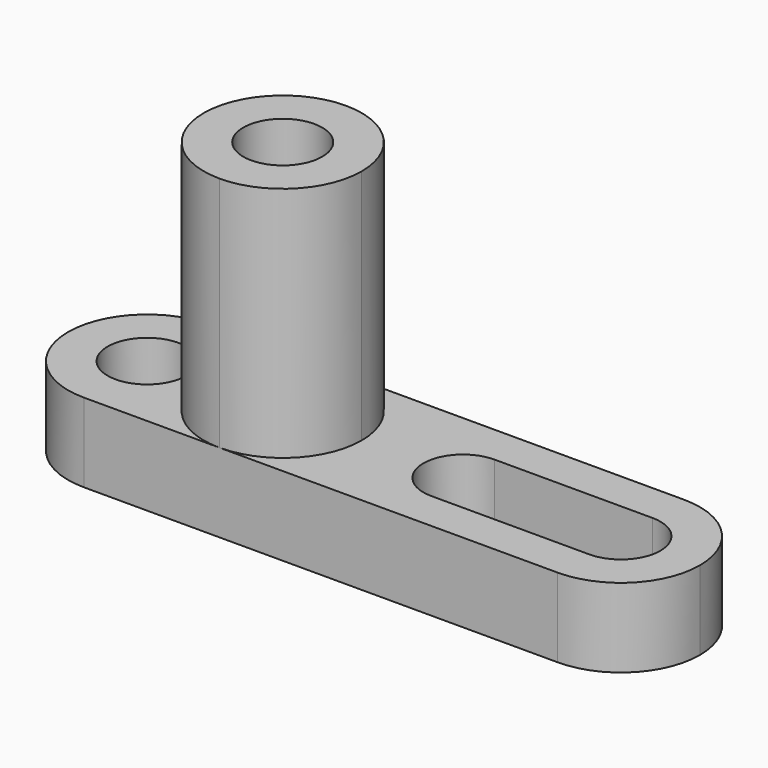
from build123d import *

# Parameters (mm, degrees)
F1_DEPTH = 25.4
F3_DEPTH = 38.1
F4_R     = 6.35
F5_DEPTH = 25.4
F7_DEPTH = 25.4
F8_R     = 6.35
F9_DEPTH = 127


# Not quite as in the source:
# - a feature names something its author has since deleted; it is built from what else it names


with BuildPart() as f1:
    # F0 (on Front) → F1 (new body)
    with BuildSketch(Plane.XZ):
        Polygon((-21.8179498348, 12.7), (-21.8179498348, 0), (79.7820501652, 0), (79.7820501652, 12.7), (25.4, 12.7), (25.4, 50.8), (0, 50.8), (0, 12.7), align=None)
    extrude(amount=F1_DEPTH)

    # F2 (on face) → F3 (cut)
    with BuildSketch(Plane.XY.offset(50.8)):
        with BuildLine():
            ThreePointArc((12.7, 0), (21.6802561211, -3.7197438789), (25.4, -12.7))
            Line((25.4, -12.7), (25.4, 0))
            Line((25.4, 0), (12.7, 0))
        make_face()
        with BuildLine():
            ThreePointArc((0, -12.7), (3.7197438789, -3.7197438789), (12.7, 0))
            Line((12.7, 0), (0, 0))
            Line((0, 0), (0, -12.7))
        make_face()
        with BuildLine():
            Line((0, -25.4), (12.7, -25.4))
            ThreePointArc((12.7, -25.4), (3.7197438789, -21.6802561211), (0, -12.7))
            Line((0, -12.7), (0, -25.4))
        make_face()
        with BuildLine():
            Line((25.4, -25.4), (25.4, -12.7))
            ThreePointArc((25.4, -12.7), (21.6802561211, -21.6802561211), (12.7, -25.4))
            Line((12.7, -25.4), (25.4, -25.4))
        make_face()
    extrude(amount=-F3_DEPTH, mode=Mode.SUBTRACT)

    # F4 (on face) → F5 (cut)
    with BuildSketch(Plane.XY.offset(12.7)):
        with Locations((-9.1179498348, -12.7)):
            Circle(F4_R)
        with BuildLine():
            ThreePointArc((-21.8179498348, -12.7), (-18.0982059559, -3.7197438789), (-9.1179498348, 0))
            Line((-9.1179498348, 0), (-21.8179498348, 0))
            Line((-21.8179498348, 0), (-21.8179498348, -12.7))
        make_face()
        with BuildLine():
            ThreePointArc((-9.1179498348, -25.4), (-18.0982059559, -21.6802561211), (-21.8179498348, -12.7))
            Line((-21.8179498348, -12.7), (-21.8179498348, -25.4))
            Line((-21.8179498348, -25.4), (-9.1179498348, -25.4))
        make_face()
    extrude(amount=-F5_DEPTH, mode=Mode.SUBTRACT)

    # F6 (on face) → F7 (cut)
    with BuildSketch(Plane.XY.offset(12.7)):
        with BuildLine():
            ThreePointArc((67.0820501652, 0), (76.0623062862, -3.7197438789), (79.7820501652, -12.7))
            Line((79.7820501652, -12.7), (79.7820501652, 0))
            Line((79.7820501652, 0), (67.0820501652, 0))
        make_face()
        with BuildLine():
            ThreePointArc((79.7820501652, -12.7), (76.0623062862, -21.6802561211), (67.0820501652, -25.4))
            Line((67.0820501652, -25.4), (79.7820501652, -25.4))
            Line((79.7820501652, -25.4), (79.7820501652, -12.7))
        make_face()
        with BuildLine():
            ThreePointArc((67.0820501652, -19.05), (71.5721782257, -17.1901280605), (73.4320501652, -12.7))
            ThreePointArc((73.4320501652, -12.7), (71.5721782257, -8.2098719395), (67.0820501652, -6.35))
            ThreePointArc((67.0820501652, -6.35), (60.7320501652, -12.7), (67.0820501652, -19.05))
        make_face()
        with BuildLine():
            ThreePointArc((67.0820501652, -19.05), (60.7320501652, -12.7), (67.0820501652, -6.35))
            Line((67.0820501652, -6.35), (41.6820501652, -6.35))
            ThreePointArc((41.6820501652, -6.35), (46.1721782257, -8.2098719395), (48.0320501652, -12.7))
            ThreePointArc((48.0320501652, -12.7), (46.1721782257, -17.1901280605), (41.6820501652, -19.05))
            Line((41.6820501652, -19.05), (67.0820501652, -19.05))
        make_face()
        with BuildLine():
            ThreePointArc((48.0320501652, -12.7), (46.1721782257, -8.2098719395), (41.6820501652, -6.35))
            ThreePointArc((41.6820501652, -6.35), (35.3320501652, -12.7), (41.6820501652, -19.05))
            ThreePointArc((41.6820501652, -19.05), (46.1721782257, -17.1901280605), (48.0320501652, -12.7))
        make_face()
    extrude(amount=-F7_DEPTH, mode=Mode.SUBTRACT)

    # F8 (on face) → F9 (cut)
    with BuildSketch(Plane.XY.offset(50.8)):
        with Locations((12.7, -12.7)):
            Circle(F8_R)
    extrude(amount=-F9_DEPTH, mode=Mode.SUBTRACT)


solid = f1.part
